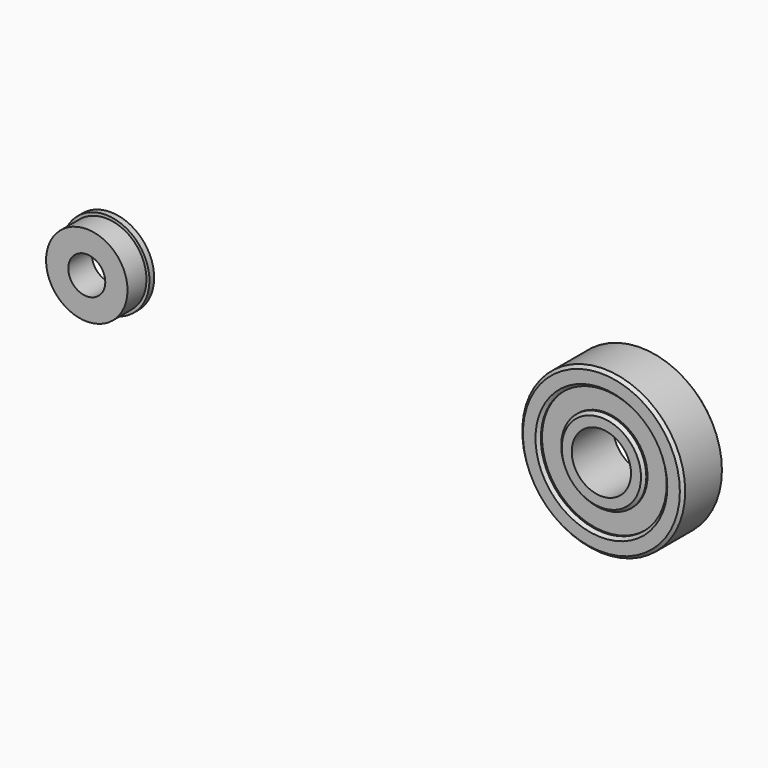
from build123d import *

# Parameters (mm, degrees)
F2_R     = 11
F2_R_2   = 4
F4_DEPTH = 3.5
F5_R     = 8.5
F5_R_2   = 5.75
F6_DEPTH = 0.6
F7_SIZE  = 0.4


# Not quite as in the source:
# - a pattern or mirror of a feature is missing from the dataset's text; its kind, count and spacing are read off the source's solid


with BuildPart() as f1:
    # F0 (on Right) → F1 (revolve)
    with BuildSketch(Plane.YZ):
        Polygon((0, 2.5), (0, 5.9), (-0.8, 5.9), (-0.8, 5.5), (-4, 5.5), (-4, 2.5), align=None)
    revolve(axis=Axis((0, -4.4890465214, 0), (0, -1, 0)))


with BuildPart() as f1_1:
    # F3: moved
    add(f1.part.moved(Location((-33.7, 0, 0))))


with BuildPart() as f4:
    # F2 (on Front) → F4 (new body, symmetric)
    with BuildSketch(Plane.XZ):
        with Locations((35.398107022, 0)):
            Circle(F2_R)
        with Locations((35.398107022, 0)):
            Circle(F2_R_2, mode=Mode.SUBTRACT)
    extrude(amount=F4_DEPTH, both=True)

    # F5 (on face) → F6 (cut)
    with BuildSketch(Plane.XZ.offset(3.5)):
        with Locations((35.398107022, 0)):
            Circle(F5_R)
        with Locations((35.398107022, 0)):
            Circle(F5_R_2, mode=Mode.SUBTRACT)
    f6 = extrude(amount=-F6_DEPTH, mode=Mode.SUBTRACT)

    # F6_copies: F6 across plane
    add(f6.mirror(Plane.ZX), mode=Mode.SUBTRACT)

    # F7
    f7_edges = [f4.edges().sort_by_distance(p)[0] for p in [
        (24.398107, -3.5, 0),
        (26.898107, -3.5, 0),
        (29.648107, -3.5, 0),
        (24.398107, 3.5, 0),
        (26.898107, 3.5, 0),
        (29.648107, 3.5, 0),
    ]]
    chamfer(f7_edges, length=F7_SIZE)


solid = Compound([f1_1.part, f4.part])
